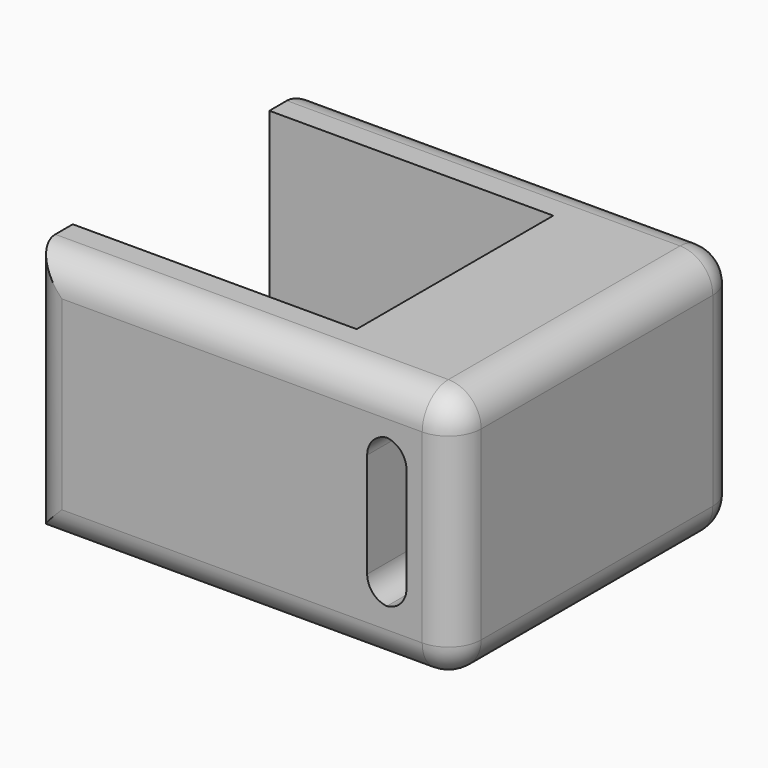
from build123d import *

# Parameters (mm, degrees)
F1_DEPTH    = 23
F2_W        = 3.6
F2_H        = 13.6
F3_DEPTH    = 48.7
F4_T1_DEPTH = 32.5
F5_R        = 3


# Not quite as in the source:
# - a fillet or chamfer that OpenCascade refuses, or shapes differently, is made with other operations: its cross-section is extruded or revolved along the edge and cut away or added


with BuildPart() as f1:
    # F0 (on Top) → F1 (new body)
    with BuildSketch(Plane.XY):
        Polygon((12.7659387215, -17.2428843321), (12.7659387215, 15.2571156679), (-26.2254474751, 15.2571156679), (-26.2254474751, 10.2571156679), (-0.2340612785, 10.2571156679), (-0.2340612785, -12.2428843321), (-26.2254474751, -12.2428843321), (-26.2254474751, -17.2428843321), align=None)
    extrude(amount=F1_DEPTH)

    # F2 (on face) → F3 (cut)
    with BuildSketch(Plane.XZ.offset(17.2428843321)):
        with Locations((6.5272997685, 11.6975279525)):
            Rectangle(F2_W, F2_H)
    extrude(amount=-F3_DEPTH, mode=Mode.SUBTRACT)

    # F4: fillet of radius 2 on 4 edges, made by hand

    # F4_s2 → F4_t1 (join)
    with BuildSketch(Plane.XZ.offset(-15.2571156679)):
        with BuildLine():
            ThreePointArc((4.7272997685, 16.4975279525), (5.3130862061, 17.9117415149), (6.7272997685, 18.4975279525))
            Line((6.7272997685, 18.4975279525), (4.7272997685, 18.4975279525))
            Line((4.7272997685, 18.4975279525), (4.7272997685, 16.4975279525))
        make_face()
        with BuildLine():
            ThreePointArc((4.7272997685, 6.8975279525), (5.3130862061, 5.4833143901), (6.7272997685, 4.8975279525))
            Line((6.7272997685, 4.8975279525), (4.7272997685, 4.8975279525))
            Line((4.7272997685, 4.8975279525), (4.7272997685, 6.8975279525))
        make_face()
        with BuildLine():
            ThreePointArc((6.3272997685, 18.4975279525), (7.7415133308, 17.9117415149), (8.3272997685, 16.4975279525))
            Line((8.3272997685, 16.4975279525), (8.3272997685, 18.4975279525))
            Line((8.3272997685, 18.4975279525), (6.3272997685, 18.4975279525))
        make_face()
        with BuildLine():
            ThreePointArc((8.3272997685, 6.8975279525), (7.7415133308, 5.4833143901), (6.3272997685, 4.8975279525))
            Line((6.3272997685, 4.8975279525), (8.3272997685, 4.8975279525))
            Line((8.3272997685, 4.8975279525), (8.3272997685, 6.8975279525))
        make_face()
    extrude(amount=F4_T1_DEPTH)

    # F5
    f5_edges = [f1.edges().sort_by_distance(p)[0] for p in [
        (-6.729754, 15.257116, 0),
        (-26.225447, 15.257116, 11.5),
        (-6.729754, 15.257116, 23),
        (-6.729754, -17.242884, 23),
        (12.765939, -0.992884, 23),
        (-6.729754, -17.242884, 0),
        (12.765939, -0.992884, 0),
        (12.765939, -17.242884, 11.5),
        (12.765939, 15.257116, 11.5),
        (-26.225447, -17.242884, 11.5),
    ]]
    fillet(f5_edges, radius=F5_R)


solid = f1.part
